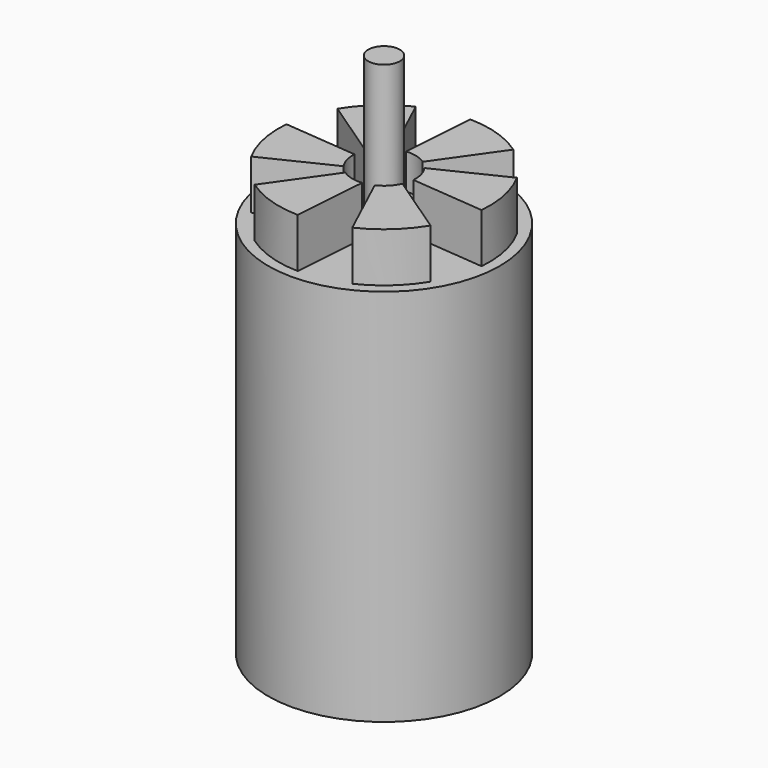
from build123d import *

# Parameters (mm, degrees)
F0_R     = 11
F1_DEPTH = 36
F2_R     = 1.5
F3_DEPTH = 1.3462
F5_R     = 1.5008527343
F6_DEPTH = 12.7
F8_DEPTH = 4.699


with BuildPart() as f1:
    # F0 (on Top) → F1 (new body)
    with BuildSketch(Plane.XY):
        Circle(F0_R)
    extrude(amount=F1_DEPTH)

    # F2 (on face) → F3 (join)
    with BuildSketch(Plane.XY.offset(36)):
        with BuildLine():
            ThreePointArc((1.7046152007, 2.4686609766), (0.7447190731, 2.906095921), (-0.3072532854, 2.984224425))
            Line((-0.3072532854, 2.984224425), (-0.3072532854, 2.2532741809))
            ThreePointArc((-0.3072532854, 2.2532741809), (-0.4284919948, 1.9952916114), (-0.704479753, 1.9239853136))
            Line((-0.704479753, 1.9239853136), (-1.2856155187, 2.7105705558))
            ThreePointArc((-1.2856155187, 2.7105705558), (-1.3939430401, 2.6564869285), (-1.5, 2.5980762114))
            ThreePointArc((-1.5, 2.5980762114), (-2.2273032861, 2.009756222), (-2.7380408053, 1.2260230619))
            Line((-2.7380408053, 1.2260230619), (-2.105019325, 0.8605479398))
            ThreePointArc((-2.105019325, 0.8605479398), (-1.9422192208, 0.6265608529), (-2.0184600346, 0.3518952942))
            Line((-2.0184600346, 0.3518952942), (-2.9902307194, 0.2419095792))
            ThreePointArc((-2.9902307194, 0.2419095792), (-2.88911243, -0.8081023245), (-2.4307875199, -1.7582013631))
            Line((-2.4307875199, -1.7582013631), (-1.7977660396, -1.392726241))
            ThreePointArc((-1.7977660396, -1.392726241), (-1.513727226, -1.3687307585), (-1.3139802816, -1.5720900194))
            Line((-1.3139802816, -1.5720900194), (-1.7046152007, -2.4686609766))
            ThreePointArc((-1.7046152007, -2.4686609766), (-0.7447190731, -2.906095921), (0.3072532854, -2.984224425))
            Line((0.3072532854, -2.984224425), (0.3072532854, -2.2532741809))
            ThreePointArc((0.3072532854, -2.2532741809), (0.4284919948, -1.9952916114), (0.704479753, -1.9239853136))
            Line((0.704479753, -1.9239853136), (1.2856155187, -2.7105705558))
            ThreePointArc((1.2856155187, -2.7105705558), (2.1443933569, -2.0979935965), (2.7380408053, -1.2260230619))
            Line((2.7380408053, -1.2260230619), (2.105019325, -0.8605479398))
            ThreePointArc((2.105019325, -0.8605479398), (1.9422192208, -0.6265608529), (2.0184600346, -0.3518952942))
            Line((2.0184600346, -0.3518952942), (2.9902307194, -0.2419095792))
            ThreePointArc((2.9902307194, -0.2419095792), (2.9975566849, -0.1210533801), (3, 0))
            ThreePointArc((3, 0), (2.8541515867, 0.9240231167), (2.4307875199, 1.7582013631))
            Line((2.4307875199, 1.7582013631), (1.7977660396, 1.392726241))
            ThreePointArc((1.7977660396, 1.392726241), (1.513727226, 1.3687307585), (1.3139802816, 1.5720900194))
            Line((1.3139802816, 1.5720900194), (1.7046152007, 2.4686609766))
        make_face()
        Circle(F2_R, mode=Mode.SUBTRACT)
    extrude(amount=F3_DEPTH)

    # F7 (on face) → F8 (join, symmetric)
    with BuildSketch(Plane.XY.offset(36)):
        with BuildLine():
            ThreePointArc((-2.4307875199, -1.7582013631), (-2.88911243, -0.8081023245), (-2.9902307194, 0.2419095792))
            Line((-2.9902307194, 0.2419095792), (-9.9625906409, 0.8641688039))
            ThreePointArc((-9.9625906409, 0.8641688039), (-9.7843590309, -2.0693330281), (-8.7596187693, -4.8238033766))
            Line((-8.7596187693, -4.8238033766), (-2.4307875199, -1.7582013631))
        make_face()
        with BuildLine():
            Line((0.2022731176, 9.99795407), (-0.3072532854, 2.984224425))
            ThreePointArc((-0.3072532854, 2.984224425), (0.7447190731, 2.906095921), (1.7046152007, 2.4686609766))
            Line((1.7046152007, 2.4686609766), (5.7296874578, 8.1957721806))
            ThreePointArc((5.7296874578, 8.1957721806), (3.1027108725, 9.5162251218), (0.2022731176, 9.99795407))
        make_face()
        with BuildLine():
            Line((8.7596187693, 4.8238033766), (2.4307875199, 1.7582013631))
            ThreePointArc((2.4307875199, 1.7582013631), (2.88911243, 0.8081023245), (2.9902307194, -0.2419095792))
            Line((2.9902307194, -0.2419095792), (9.9625906409, -0.8641688039))
            ThreePointArc((9.9625906409, -0.8641688039), (9.7892625878, 2.0703701008), (8.7596187693, 4.8238033766))
        make_face()
        with BuildLine():
            Line((8.5573456517, -5.1741506934), (2.7380408053, -1.2260230619))
            ThreePointArc((2.7380408053, -1.2260230619), (2.1443933569, -2.0979935965), (1.2856155187, -2.7105705558))
            Line((1.2856155187, -2.7105705558), (4.2329031831, -9.0599409845))
            ThreePointArc((4.2329031831, -9.0599409845), (6.6811343516, -7.4353423534), (8.5573456517, -5.1741506934))
        make_face()
        with BuildLine():
            ThreePointArc((-2.7380408053, 1.2260230619), (-2.1443933569, 2.0979935965), (-1.2856155187, 2.7105705558))
            Line((-1.2856155187, 2.7105705558), (-4.2329031831, 9.0599409845))
            ThreePointArc((-4.2329031831, 9.0599409845), (-6.6822968499, 7.4366360818), (-8.5573456517, 5.1741506934))
            Line((-8.5573456517, 5.1741506934), (-2.7380408053, 1.2260230619))
        make_face()
        with BuildLine():
            ThreePointArc((0.3072532854, -2.984224425), (-0.7447190731, -2.906095921), (-1.7046152007, -2.4686609766))
            Line((-1.7046152007, -2.4686609766), (-5.7296874578, -8.1957721806))
            ThreePointArc((-5.7296874578, -8.1957721806), (-3.1010075693, -9.5110009752), (-0.2022731176, -9.99795407))
            Line((-0.2022731176, -9.99795407), (0.3072532854, -2.984224425))
        make_face()
    extrude(amount=F8_DEPTH, both=True)


with BuildPart() as f6:
    # F5 (on face) → F6 (new body)
    with BuildSketch(Plane.XY.offset(37.3462)):
        Circle(F5_R)
    extrude(amount=F6_DEPTH)


solid = Compound([f1.part, f6.part])
